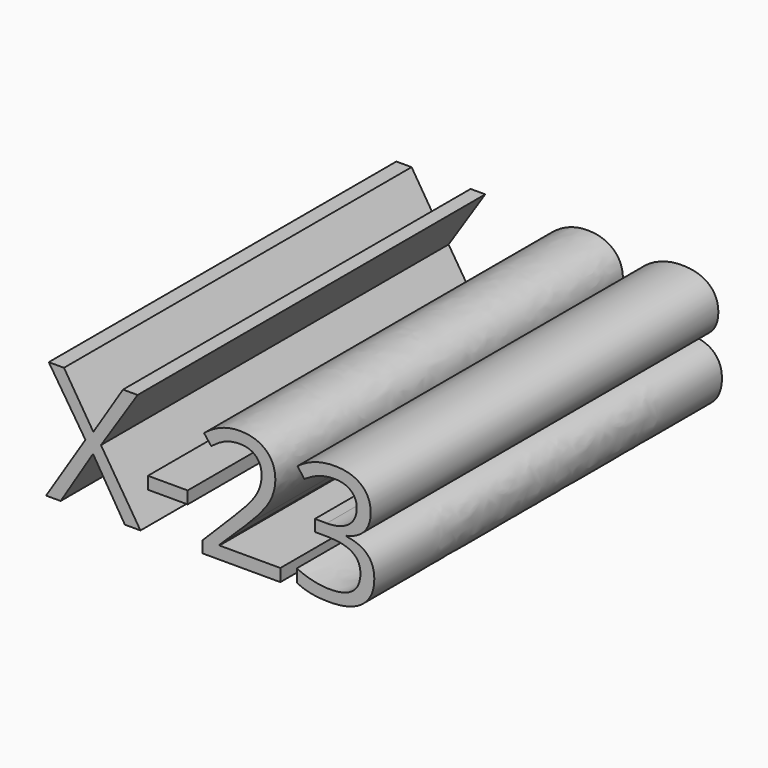
from build123d import *

# Parameters (mm, degrees)
F0_TEXT_SIZE = 48.4526066834
F1_DEPTH     = 127


# Not quite as in the source:
# - Text() gives the source's letters only with a copy of the font that has no kerning and outlines rounded to 1/6400 em; it was checked with that copy


with BuildPart() as f1:
    # F0 (on Front) → F1 (new body)
    with BuildSketch(Plane.XZ):
        with Locations((-35.7390642166, 9.3850595877)):
            Text('X-23', F0_TEXT_SIZE, font='Open Sans', text_align=(TextAlign.LEFT, TextAlign.BOTTOM))
    extrude(amount=F1_DEPTH)


solid = f1.part
